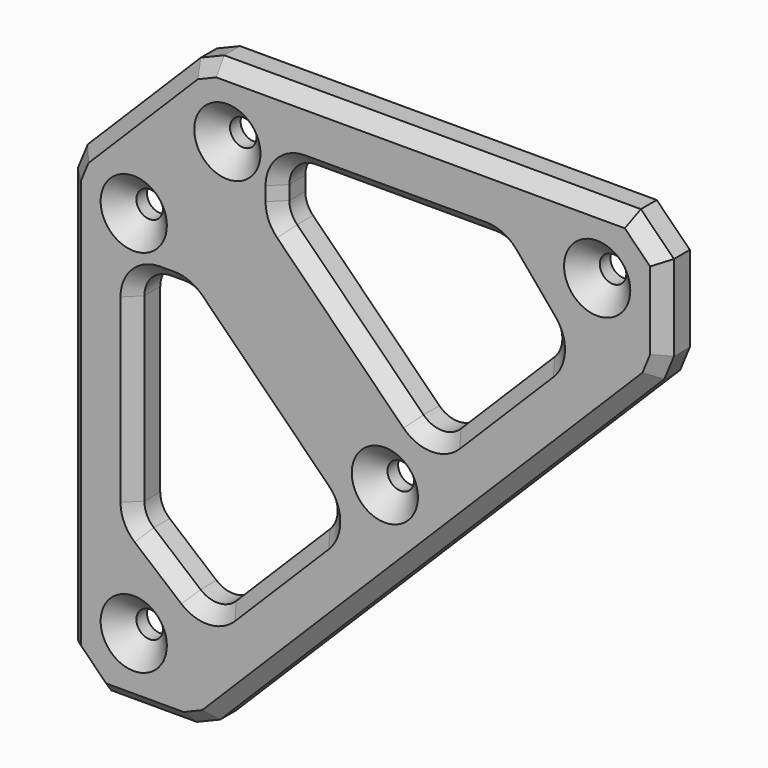
from build123d import *

# Parameters (mm, degrees)
F0_R        = 2
F1_DEPTH    = 5
F2_T1_DEPTH = 30.7168298797
F2_T3_DEPTH = 16.2857086021
F3_SIZE     = 2
F4_SIZE     = 3
F5_SIZE     = 2


# Not quite as in the source:
# - a fillet or chamfer that OpenCascade refuses, or shapes differently, is made with other operations: its cross-section is extruded or revolved along the edge and cut away or added


with BuildPart() as f1:
    # F0 (on Front) → F1 (new body)
    with BuildSketch(Plane.XZ):
        Polygon((20, 0), (0, -20), (0, -90), (20, -90), (90, -20), (90, 0), align=None)
        with Locations((10, -80)):
            Circle(F0_R, mode=Mode.SUBTRACT)
        with BuildLine():
            Line((14, -31.908116908), (16.1091270347, -31.908116908))
            ThreePointArc((16.1091270347, -31.908116908), (17.6398607642, -32.2125987779), (18.9375541595, -33.0796897832))
            Line((18.9375541595, -33.0796897832), (38.0294372515, -52.1715728753))
            ThreePointArc((38.0294372515, -52.1715728753), (39.2010101268, -55), (38.0294372515, -57.8284271247))
            Line((38.0294372515, -57.8284271247), (23.8873016278, -71.9705627485))
            ThreePointArc((23.8873016278, -71.9705627485), (21.2333520525, -73.1383285101), (18.4877240643, -72.2063133962))
            Line((18.4877240643, -72.2063133962), (11.4288495613, -66.2832144042))
            ThreePointArc((11.4288495613, -66.2832144042), (10.3747688519, -64.9095096787), (10, -63.2190366317))
            Line((10, -63.2190366317), (10, -35.908116908))
            ThreePointArc((10, -35.908116908), (11.1715728753, -33.0796897832), (14, -31.908116908))
        make_face(mode=Mode.SUBTRACT)
        with Locations((47.9289321881, -47.9289321881)):
            Circle(F0_R, mode=Mode.SUBTRACT)
        with Locations((10, -24.1421356237)):
            Circle(F0_R, mode=Mode.SUBTRACT)
        with Locations((24.1421356237, -10)):
            Circle(F0_R, mode=Mode.SUBTRACT)
        with BuildLine():
            ThreePointArc((63.2190366317, -10), (64.9095096787, -10.3747688519), (66.2832144042, -11.4288495613))
            Line((66.2832144042, -11.4288495613), (72.2063133962, -18.4877240643))
            ThreePointArc((72.2063133962, -18.4877240643), (73.1383285101, -21.2333520525), (71.9705627485, -23.8873016278))
            Line((71.9705627485, -23.8873016278), (57.8284271247, -38.0294372515))
            ThreePointArc((57.8284271247, -38.0294372515), (55, -39.2010101268), (52.1715728753, -38.0294372515))
            Line((52.1715728753, -38.0294372515), (33.0796897832, -18.9375541595))
            ThreePointArc((33.0796897832, -18.9375541595), (32.2125987779, -17.6398607642), (31.908116908, -16.1091270347))
            Line((31.908116908, -16.1091270347), (31.908116908, -14))
            ThreePointArc((31.908116908, -14), (33.0796897832, -11.1715728753), (35.908116908, -10))
            Line((35.908116908, -10), (63.2190366317, -10))
        make_face(mode=Mode.SUBTRACT)
        with Locations((80, -10)):
            Circle(F0_R, mode=Mode.SUBTRACT)
    extrude(amount=F1_DEPTH)

    # F2: chamfer of 5 on 6 edges, made by hand

    # F2_s2 → F2_t1 (cut)
    with BuildSketch(Plane.XZ.offset(-12.8584149398)):
        Polygon((90, -5), (85, 0), (90, 0), align=None)
        Polygon((0, -85), (5, -90), (0, -90), align=None)
    extrude(amount=F2_T1_DEPTH, mode=Mode.SUBTRACT)

    # F2_s4 → F2_t3 (cut)
    with BuildSketch(Plane.XZ.offset(-5.6428543011)):
        Polygon((1.4644660941, -18.5355339059), (0, -22.0710678119), (0, -20), align=None)
        Polygon((18.5355339059, -1.4644660941), (22.0710678119, 0), (20, 0), align=None)
        Polygon((88.5355339059, -21.4644660941), (90, -17.9289321881), (90, -20), align=None)
        Polygon((17.9289321881, -90), (21.4644660941, -88.5355339059), (20, -90), align=None)
    extrude(amount=F2_T3_DEPTH, mode=Mode.SUBTRACT)

    # F3
    f3_edges = [f1.edges().sort_by_distance(p)[0] for p in [
        (0.732233, -5, -20.303301),
        (20.303301, -5, -0.732233),
        (10, -5, -10),
        (87.5, -5, -2.5),
        (89.267767, -5, -19.696699),
        (90, -5, -11.464466),
        (53.535534, -5, 0),
        (19.696699, -5, -89.267767),
        (2.5, -5, -87.5),
        (11.464466, -5, -90),
        (0, -5, -53.535534),
        (55, -5, -55),
    ]]
    chamfer(f3_edges, length=F3_SIZE)

    # F4
    f4_edges = [f1.edges().sort_by_distance(p)[0] for p in [
        (8, -5, -24.142136),
        (22.142136, -5, -10),
        (78, -5, -10),
        (45.928932, -5, -47.928932),
        (8, -5, -80),
    ]]
    chamfer(f4_edges, length=F4_SIZE)

    # F5
    f5_edges = [f1.edges().sort_by_distance(p)[0] for p in [
        (30.958369, -5, -64.899495),
        (21.233352, -5, -73.138329),
        (14.958287, -5, -69.244764),
        (10.374769, -5, -64.90951),
        (10, -5, -49.563577),
        (11.171573, -5, -33.07969),
        (17.639861, -5, -32.212599),
        (14, -2.5, -31.908117),
        (15.054564, -5, -31.908117),
        (28.483496, -5, -42.625631),
        (39.20101, -5, -55),
        (42.625631, -5, -28.483496),
        (33.07969, -5, -11.171573),
        (31.908117, -5, -15.054564),
        (49.563577, -5, -10),
        (32.212599, -5, -17.639861),
        (64.90951, -5, -10.374769),
        (69.244764, -5, -14.958287),
        (55, -5, -39.20101),
        (73.138329, -5, -21.233352),
        (64.899495, -5, -30.958369),
    ]]
    chamfer(f5_edges, length=F5_SIZE)


solid = f1.part
